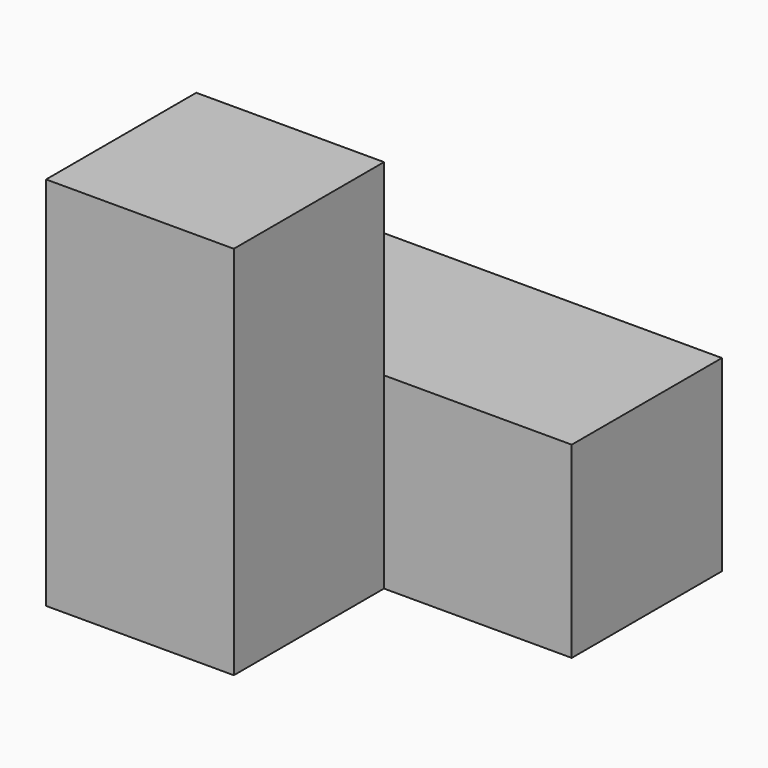
from build123d import *

# Parameters (mm, degrees)
F1_W     = 50.8
F1_H     = 50.8
F2_DEPTH = 25.4
F3_W     = 25.4
F3_H     = 25.4
F4_DEPTH = 25.4
F5_W     = 25.4
F5_H     = 25.4
F6_DEPTH = 25.4


# Not quite as in the source:
# - a variable given as a bare number and used for a length is read in inches; the dataset says mm whatever the document's units were


with BuildPart() as f2:
    # F1 (on Top) → F2 (new body)
    with BuildSketch(Plane.XY):
        Rectangle(F1_W, F1_H)
    extrude(amount=F2_DEPTH)

    # F3 (on face) → F4 (cut)
    with BuildSketch(Plane.XY.offset(25.4)):
        with Locations((12.7, -12.7)):
            Rectangle(F3_W, F3_H)
    extrude(amount=-F4_DEPTH, mode=Mode.SUBTRACT)

    # F5 (on face) → F6 (join)
    with BuildSketch(Plane.XY.offset(25.4)):
        with Locations((-12.7, -12.7)):
            Rectangle(F5_W, F5_H)
    extrude(amount=F6_DEPTH)


solid = f2.part
